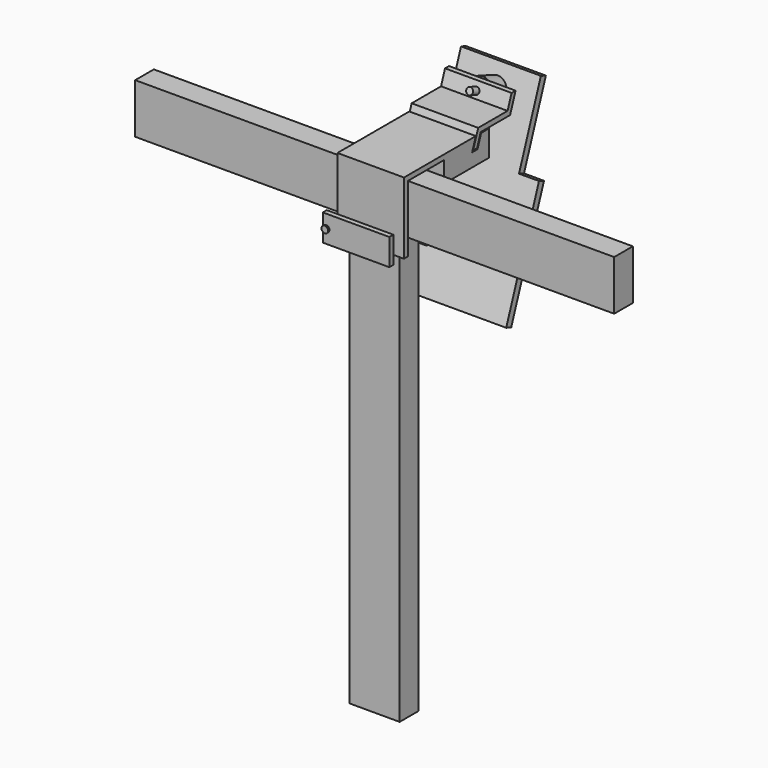
from build123d import *

# Parameters (mm, degrees)
F1_DEPTH  = 47.625
F2_DEPTH  = 457.2
F3_DEPTH  = 63.5
F0_W      = 9.525
F0_H      = 50.8
F4_DEPTH  = 63.5
F5_R      = 6.35
F6_DEPTH  = 38.1
F7_W      = 152.4
F7_H      = 152.4
F8_DEPTH  = 12.7
F9_DEPTH  = 76.2
F10_R     = 9.525
F10_R_2   = 6.35
F11_DEPTH = 3.175
F12_DEPTH = 76.2
F13_R     = 3.175
F14_DEPTH = 127
F15_DEPTH = 114.3
F16_DEPTH = 3.175


with BuildPart() as f1:
    # F0 (on Right) → F1 (new body, symmetric)
    with BuildSketch(Plane.YZ):
        Polygon((0, -95.25), (-44.45, -95.25), (-44.45, -127), (-44.45, -914.4), (0, -914.4), (0, -127), align=None)
    extrude(amount=F1_DEPTH, both=True)

    # F0 (on Right) → F2 (join, symmetric)
    with BuildSketch(Plane.YZ):
        Polygon((0, 0), (-44.45, 0), (-44.45, -95.25), (0, -95.25), (0, -76.2), align=None)
    extrude(amount=F2_DEPTH, both=True)


with BuildPart() as f3:
    # F0 (on Right) → F3 (new body, symmetric)
    with BuildSketch(Plane.YZ):
        Polygon((-44.45, -95.25), (-44.45, 0), (-53.975, 0), (-53.975, -127), (-44.45, -127), align=None)
        Polygon((-53.975, 0), (-44.45, 0), (0, 0), (41.275, 0), (114.0081835186, 0), (117.475, 9.525), (-53.975, 9.525), align=None)
        Polygon((114.0081835186, 0), (41.275, 0), (41.275, -39.751), (149.225, -39.751), (149.225, 0), (126.7081835186, 0), (121.4848466867, -14.351), (108.7848466867, -14.351), align=None)
        Polygon((126.7081835186, 0), (149.225, 0), (149.225, 9.525), (130.175, 9.525), align=None)
    extrude(amount=F3_DEPTH, both=True)


with BuildPart() as f3b:
    # F0 (on Right) → F3, piece 2 (new body, symmetric)
    with BuildSketch(Plane.YZ):
        Polygon((9.525, -76.2), (0, -76.2), (0, -95.25), (0, -127), (9.525, -127), align=None)
    extrude(amount=F3_DEPTH, both=True)


with BuildPart() as f3c:
    # F0 (on Right) → F3, piece 3 (new body, symmetric)
    with BuildSketch(Plane.YZ):
        with Locations((-84.1375, -101.6)):
            Rectangle(F0_W, F0_H)
    extrude(amount=F3_DEPTH, both=True)


with BuildPart() as f4:
    # F0 (on Right) → F4 (new body, symmetric)
    with BuildSketch(Plane.YZ):
        Polygon((202.8391554729, 47.2850536329), (193.2750044936, 21.0077647809), (199.3331880122, 21.0077647809), (199.3331880122, 11.4827647809), (212.3641554729, 47.2850536329), align=None)
        Polygon((199.3331880122, 21.0077647809), (193.2750044936, 21.0077647809), (189.8081880122, 11.4827647809), (199.3331880122, 11.4827647809), align=None)
        Polygon((132.6581880122, 21.0077647809), (129.1913715308, 11.4827647809), (130.887568106, 11.4827647809), (134.3543845873, 21.0077647809), align=None)
        Polygon((132.6581880122, 21.0077647809), (123.1331880122, 21.0077647809), (123.1331880122, 11.4827647809), (129.1913715308, 11.4827647809), align=None)
        Polygon((123.1331880122, 21.0077647809), (118.9538034249, 9.525), (128.4788034249, 9.525), (129.1913715308, 11.4827647809), (123.1331880122, 11.4827647809), align=None)
        Polygon((118.9538034249, 9.525), (115.4869869435, 0), (125.0119869435, 0), (128.4788034249, 9.525), align=None)
        Polygon((125.0119869435, 0), (115.4869869435, 0), (111.1881345066, -11.811), (120.7131345066, -11.811), align=None)
        Polygon((193.2750044936, 21.0077647809), (134.3543845873, 21.0077647809), (130.887568106, 11.4827647809), (189.8081880122, 11.4827647809), align=None)
    extrude(amount=F4_DEPTH, both=True)


with BuildPart() as f6:
    # F5 (on face) → F6 (new body)
    with BuildSketch(Plane(origin=(0, 172.325145046, -62.7212234124), x_dir=(-1, 0, 0), z_dir=(0, 0.9396926208, -0.3420201433))):
        with BuildLine():
            ThreePointArc((11.4476252996, 78.9662348644), (19.3439150288, 87.0725802482), (22.225, 98.0162348644))
            ThreePointArc((22.225, 98.0162348644), (19.3439150288, 108.9598894806), (11.4476252996, 117.0662348644))
            Line((11.4476252996, 117.0662348644), (-11.4476252996, 117.0662348644))
            ThreePointArc((-11.4476252996, 117.0662348644), (-22.225, 98.0162348644), (-11.4476252996, 78.9662348644))
            Line((-11.4476252996, 78.9662348644), (11.4476252996, 78.9662348644))
        make_face()
        with Locations((0, 98.0162348644)):
            Circle(F5_R, mode=Mode.SUBTRACT)
        with Locations((0, 98.0162348644)):
            Circle(F5_R)
        with BuildLine():
            Line((-11.4476252996, 117.0662348644), (11.4476252996, 117.0662348644))
            ThreePointArc((11.4476252996, 117.0662348644), (0, 120.2412348644), (-11.4476252996, 117.0662348644))
        make_face()
        with BuildLine():
            ThreePointArc((-11.4476252996, 78.9662348644), (0, 75.7912348644), (11.4476252996, 78.9662348644))
            Line((11.4476252996, 78.9662348644), (-11.4476252996, 78.9662348644))
        make_face()
    extrude(amount=F6_DEPTH)


with BuildPart() as f8:
    # F7 (on face) → F8 (new body)
    with BuildSketch(Plane(origin=(0, 208.127433898, -75.7521908731), x_dir=(-1, 0, 0), z_dir=(0, 0.9396926208, -0.3420201433))):
        Polygon((114.3, -9.9337651356), (76.2, -9.9337651356), (-76.2, -9.9337651356), (-114.3, -9.9337651356), (-114.3, -238.5337651356), (114.3, -238.5337651356), align=None)
        with Locations((0, 66.2662348644)):
            Rectangle(F7_W, F7_H)
    extrude(amount=F8_DEPTH)


with BuildPart() as f9_tool:
    # F5 (on face) → F9 (new body, symmetric)
    with BuildSketch(Plane(origin=(0, 172.325145046, -62.7212234124), x_dir=(-1, 0, 0), z_dir=(0, 0.9396926208, -0.3420201433))):
        with Locations((0, 98.0162348644)):
            Circle(F5_R)
    extrude(amount=F9_DEPTH, both=True)


with BuildPart() as f4_1:
    add(f4.part)

    # F9: cut by f9_tool
    add(f9_tool.part, mode=Mode.SUBTRACT)


with BuildPart() as f6_1:
    add(f6.part)

    # F9: cut by f9_tool
    add(f9_tool.part, mode=Mode.SUBTRACT)


with BuildPart() as f8_1:
    add(f8.part)

    # F9: cut by f9_tool
    add(f9_tool.part, mode=Mode.SUBTRACT)


with BuildPart() as f11:
    # F10 (on face) → F11 (new body)
    with BuildSketch(Plane(origin=(0, 220.0615301819, -80.0958466933), x_dir=(-1, 0, 0), z_dir=(0, 0.9396926208, -0.3420201433))):
        with Locations((0, 98.0162348644)):
            Circle(F10_R)
        with Locations((0, 98.0162348644)):
            Circle(F10_R_2, mode=Mode.SUBTRACT)
        with Locations((0, 98.0162348644)):
            Circle(F10_R_2)
    extrude(amount=F11_DEPTH)

    # F10 (on face) → F12 (join)
    with BuildSketch(Plane(origin=(0, 220.0615301819, -80.0958466933), x_dir=(-1, 0, 0), z_dir=(0, 0.9396926208, -0.3420201433))):
        with Locations((0, 98.0162348644)):
            Circle(F10_R_2)
    extrude(amount=-F12_DEPTH)


with BuildPart() as f14_tool:
    # F13 (on face) → F14 (new body)
    with BuildSketch(Plane.XZ.offset(88.9)):
        with Locations((-57.15, -101.6)):
            Circle(F13_R)
    extrude(amount=-F14_DEPTH)


with BuildPart() as f3_1:
    add(f3.part)

    # F14: cut by f14_tool
    add(f14_tool.part, mode=Mode.SUBTRACT)


with BuildPart() as f3b_1:
    add(f3b.part)

    # F14: cut by f14_tool
    add(f14_tool.part, mode=Mode.SUBTRACT)


with BuildPart() as f3c_1:
    add(f3c.part)

    # F14: cut by f14_tool
    add(f14_tool.part, mode=Mode.SUBTRACT)


with BuildPart() as f15:
    # F13 (on face) → F15 (new body)
    with BuildSketch(Plane.XZ.offset(88.9)):
        with Locations((-57.15, -101.6)):
            Circle(F13_R)
    extrude(amount=-F15_DEPTH)

    # F13 (on face) → F16 (join)
    with BuildSketch(Plane.XZ.offset(88.9)):
        with BuildLine():
            ThreePointArc((-63.5, -101.6), (-57.15, -107.95), (-50.8, -101.6))
            ThreePointArc((-50.8, -101.6), (-57.15, -95.25), (-63.5, -101.6))
        make_face()
        with Locations((-57.15, -101.6)):
            Circle(F13_R, mode=Mode.SUBTRACT)
        with Locations((-57.15, -101.6)):
            Circle(F13_R)
    extrude(amount=F16_DEPTH)


solid = Compound([f1.part, f4_1.part, f6_1.part, f8_1.part, f11.part, f3_1.part, f3b_1.part, f3c_1.part, f15.part])
